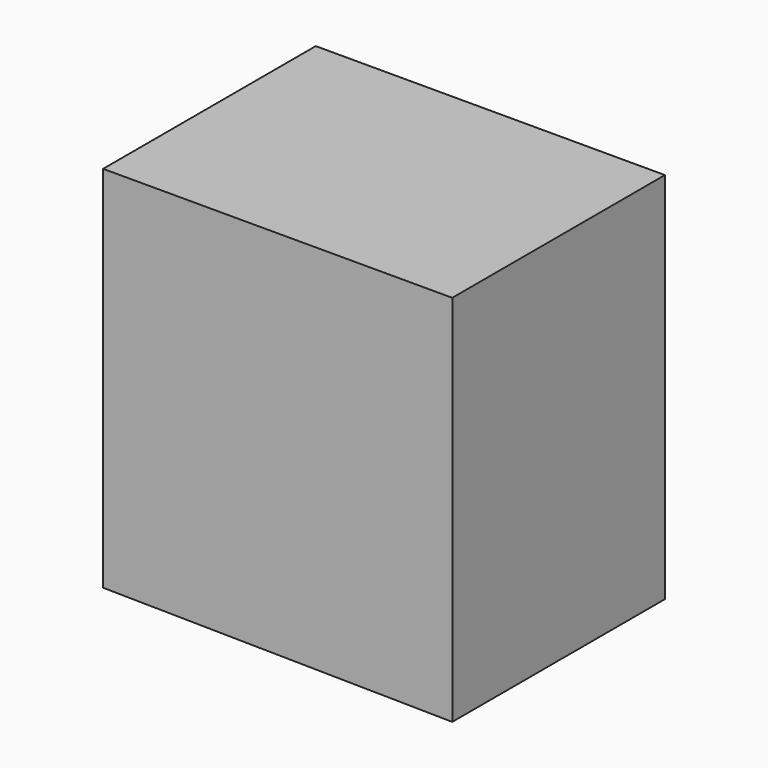
from build123d import *

# Parameters (mm, degrees)
F2_DEPTH = 80.3967639804


# Not quite as in the source:
# - the program builds the solid bodies; features that only make, move or delete a surface that nothing else refers to are left out


with BuildPart() as f2:
    # F0 (on Front) → F2 (new body)
    with BuildSketch(Plane.XZ):
        Polygon((-46.0283830762, 59.7869642079), (-46.0283830762, -51.7659522593), (59.5810115337, -53.1484037638), (59.5810115337, 59.7869642079), align=None)
    extrude(amount=F2_DEPTH)


solid = f2.part
